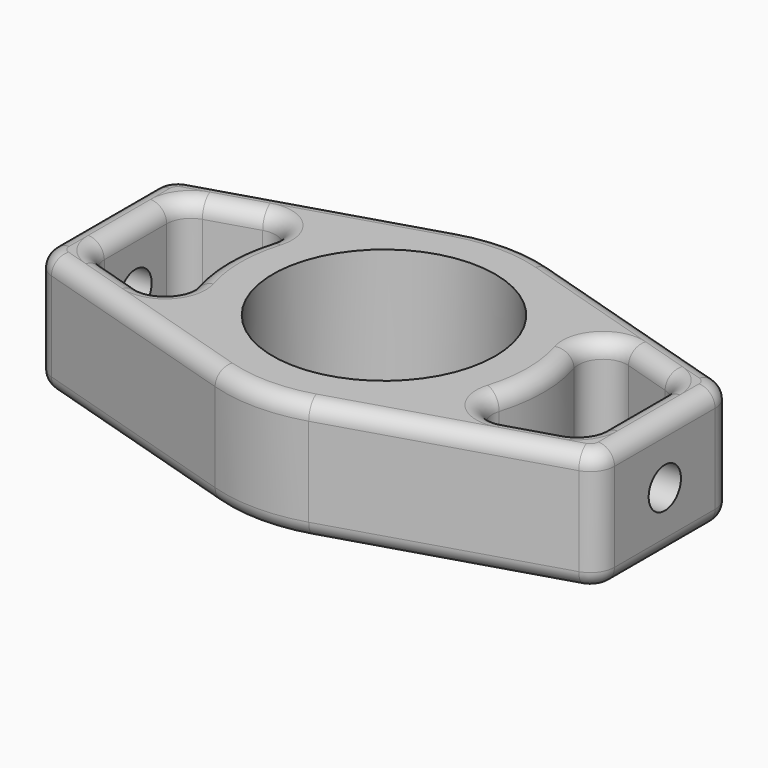
from build123d import *

# Parameters (mm, degrees)
F0_R      = 13.75
F1_DEPTH  = 15
F2_R      = 3
F3_R      = 3
F4_R      = 3
F5_R      = 3
F6_R      = 2
F7_R      = 2
F8_R      = 1.99999
F9_R      = 1.99999
F10_R     = 1.99999
F11_R     = 1.99999
F12_R     = 2.5
F13_DEPTH = 5
F14_R     = 2.5
F15_DEPTH = 5


# Not quite as in the source:
# - a fillet or chamfer is up to 0.001 mm smaller than in the source, because OpenCascade refuses the exact size


with BuildPart() as f1:
    # F0 (on Top) → F1 (new body)
    with BuildSketch(Plane.XY):
        with BuildLine():
            Line((-34.75, 10), (-34.75, -10))
            Line((-34.75, -10), (-5.7911916553, -18.8818589978))
            ThreePointArc((-5.7911916553, -18.8818589978), (0, -19.75), (5.7911916553, -18.8818589978))
            Line((5.7911916553, -18.8818589978), (34.75, -10))
            Line((34.75, -10), (34.75, 10))
            Line((34.75, 10), (5.7911916553, 18.8818589978))
            ThreePointArc((5.7911916553, 18.8818589978), (0, 19.75), (-5.7911916553, 18.8818589978))
            Line((-5.7911916553, 18.8818589978), (-34.75, 10))
        make_face()
        with BuildLine():
            Line((16.0108651403, 11.5635071436), (30.75, 7.0429165166))
            Line((30.75, 7.0429165166), (30.75, -7.0429165166))
            Line((30.75, -7.0429165166), (16.0108651403, -11.5635071436))
            ThreePointArc((16.0108651403, -11.5635071436), (19.75, 0), (16.0108651403, 11.5635071436))
        make_face(mode=Mode.SUBTRACT)
        with BuildLine():
            Line((-30.75, 7.0429165166), (-16.0108651403, 11.5635071436))
            ThreePointArc((-16.0108651403, 11.5635071436), (-19.75, 0), (-16.0108651403, -11.5635071436))
            Line((-16.0108651403, -11.5635071436), (-30.75, -7.0429165166))
            Line((-30.75, -7.0429165166), (-30.75, 7.0429165166))
        make_face(mode=Mode.SUBTRACT)
        Circle(F0_R, mode=Mode.SUBTRACT)
    extrude(amount=F1_DEPTH)

    # F2
    f2_edges = [f1.edges().sort_by_distance(p)[0] for p in [
        (-30.75, 7.042917, 7.5),
        (-30.75, -7.042917, 7.5),
        (-16.010865, 11.563507, 7.5),
        (-16.010865, -11.563507, 7.5),
    ]]
    fillet(f2_edges, radius=F2_R)

    # F3
    f3_edges = [f1.edges().sort_by_distance(p)[0] for p in [
        (16.010865, 11.563507, 7.5),
        (30.75, 7.042917, 7.5),
        (30.75, -7.042917, 7.5),
        (16.010865, -11.563507, 7.5),
    ]]
    fillet(f3_edges, radius=F3_R)

    # F4
    f4_edges = [f1.edges().sort_by_distance(p)[0] for p in [
        (34.75, -10, 7.5),
        (34.75, 10, 7.5),
    ]]
    fillet(f4_edges, radius=F4_R)

    # F5
    f5_edges = [f1.edges().sort_by_distance(p)[0] for p in [
        (-34.75, 10, 7.5),
        (-34.75, -10, 7.5),
    ]]
    fillet(f5_edges, radius=F5_R)

    # F6
    f6_edges = [f1.edges().sort_by_distance(p)[0] for p in [
        (-19.210433, 14.766088, 15),
    ]]
    fillet(f6_edges, radius=F6_R)

    # F7
    f7_edges = [f1.edges().sort_by_distance(p)[0] for p in [
        (-19.210433, -14.766088, 0),
    ]]
    fillet(f7_edges, radius=F7_R)

    # F8 (radius 2 in the source; OpenCascade refuses exactly that, so slightly less here)
    f8_edges = [f1.edges().sort_by_distance(p)[0] for p in [
        (-25.630603, 8.61307, 15),
    ]]
    fillet(f8_edges, radius=F8_R)

    # F9 (radius 2 in the source; OpenCascade refuses exactly that, so slightly less here)
    f9_edges = [f1.edges().sort_by_distance(p)[0] for p in [
        (25.630603, 8.61307, 15),
    ]]
    fillet(f9_edges, radius=F9_R)

    # F10 (radius 2 in the source; OpenCascade refuses exactly that, so slightly less here)
    f10_edges = [f1.edges().sort_by_distance(p)[0] for p in [
        (-25.630603, -8.61307, 0),
    ]]
    fillet(f10_edges, radius=F10_R)

    # F11 (radius 2 in the source; OpenCascade refuses exactly that, so slightly less here)
    f11_edges = [f1.edges().sort_by_distance(p)[0] for p in [
        (25.630603, -8.61307, 0),
    ]]
    fillet(f11_edges, radius=F11_R)

    # F12 (on face) → F13 (cut)
    with BuildSketch(Plane(origin=(-34.75, 0, 0), x_dir=(0, -1, 0), z_dir=(-1, 0, 0))):
        with Locations((0, 7.5)):
            Circle(F12_R)
    extrude(amount=-F13_DEPTH, mode=Mode.SUBTRACT)

    # F14 (on face) → F15 (cut)
    with BuildSketch(Plane.YZ.offset(34.75)):
        with Locations((0, 7.5)):
            Circle(F14_R)
    extrude(amount=-F15_DEPTH, mode=Mode.SUBTRACT)


solid = f1.part
